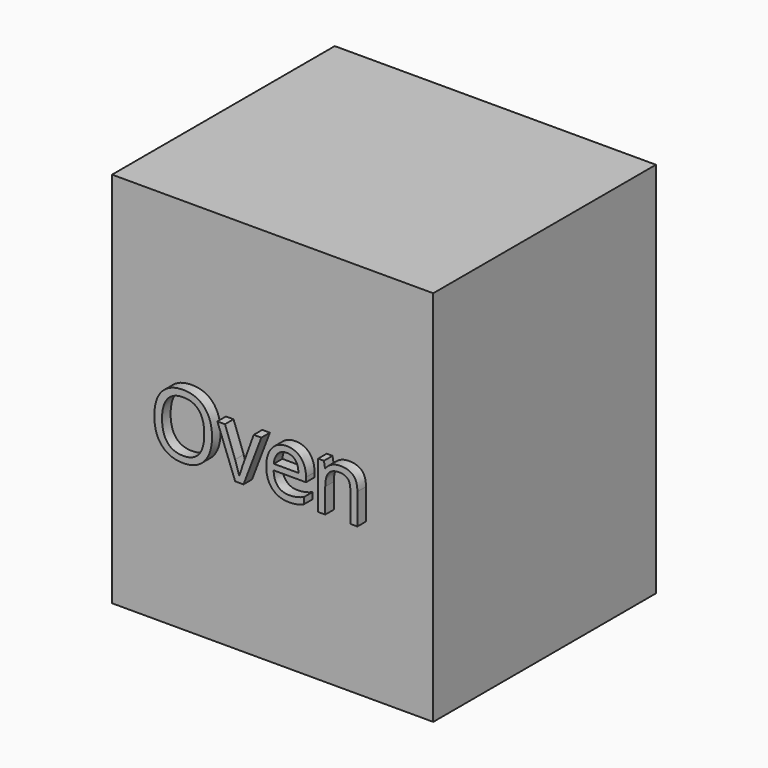
from build123d import *

# Parameters (mm, degrees)
F0_W         = 762
F0_H         = 895.35
F1_DEPTH     = 660.4
F2_TEXT_SIZE = 208.2900890512
F3_DEPTH     = 25.4


# Not quite as in the source:
# - Text() gives the source's letters only with a copy of the font that has no kerning and outlines rounded to 1/6400 em; it was checked with that copy


with BuildPart() as f1:
    # F0 (on Front) → F1 (new body)
    with BuildSketch(Plane.XZ):
        with Locations((-381, 447.675)):
            Rectangle(F0_W, F0_H)
    extrude(amount=F1_DEPTH)

    # F2 (on face) → F3 (join)
    with BuildSketch(Plane.XZ.offset(660.4)):
        with Locations((-654.1257038159, 366.6000928257)):
            Text('Oven', F2_TEXT_SIZE, font='Open Sans', text_align=(TextAlign.LEFT, TextAlign.BOTTOM))
    extrude(amount=F3_DEPTH)


solid = f1.part
